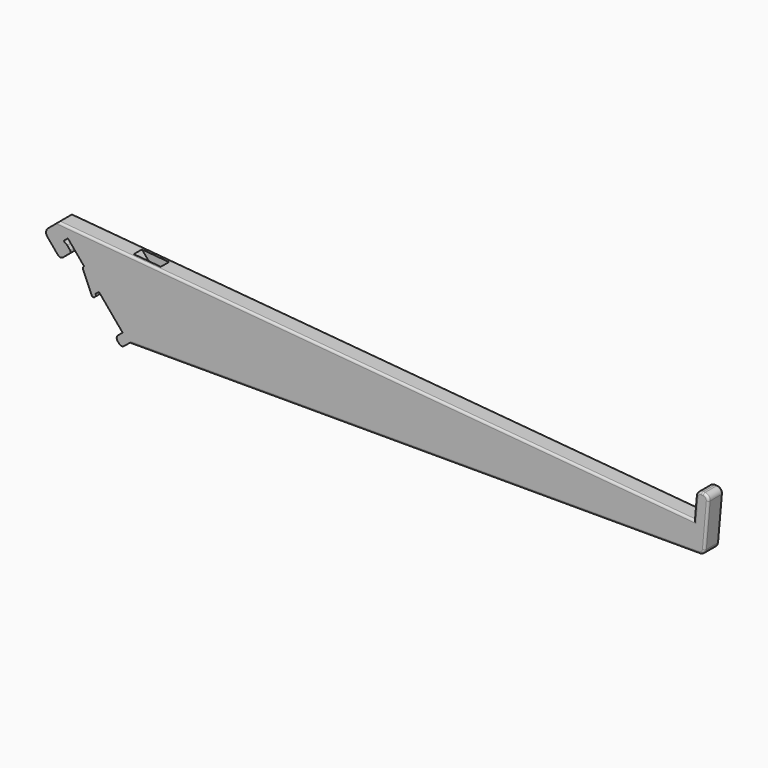
from build123d import *

# Parameters (mm, degrees)
F1_DEPTH = 12.7
F2_W     = 13.335
F2_H     = 7.112
F3_DEPTH = 93.472
F5_R     = 1.524


# Not quite as in the source:
# - two fillets or chamfers of one size are made in one step


with BuildPart() as f1:
    # F0 (on Front) → F1 (new body)
    with BuildSketch(Plane.XZ):
        with BuildLine():
            ThreePointArc((-46.0617865298, -15.3783926414), (-47.4082675367, -17.9649585898), (-46.5313950652, -20.7460427626))
            Line((-46.5313950652, -20.7460427626), (-39.1843326865, -29.5019307475))
            ThreePointArc((-39.1843326865, -29.5019307475), (-37.4599553875, -30.399584752), (-35.6058992724, -29.8150031044))
            Line((-35.6058992724, -29.8150031044), (-30.7415170586, -25.7333017829))
            ThreePointArc((-30.7415170586, -25.7333017829), (-30.2926900563, -24.8711131334), (-30.5849808801, -23.9440850758))
            Line((-30.5849808801, -23.9440850758), (-32.6258315409, -21.5118939689))
            Line((-32.6258315409, -21.5118939689), (-35.2214163384, -19.5451800716))
            Line((-35.2214163384, -19.5451800716), (-32.2344910947, -17.0388522013))
            Line((-32.2344910947, -17.0388522013), (-20.8873614209, -30.5618347556))
            Line((-20.8873614209, -30.5618347556), (-21.3737996423, -30.9700048878))
            ThreePointArc((-21.3737996423, -30.9700048878), (-21.7934146066, -31.6507945747), (-21.722945379, -32.4474032641))
            Line((-21.722945379, -32.4474032641), (-15.4658563045, -46.9017792559))
            ThreePointArc((-15.4658563045, -46.9017792559), (-14.603667655, -47.3506062582), (-13.6766395974, -47.0583154344))
            Line((-13.6766395974, -47.0583154344), (-12.2173249333, -45.8338050379))
            Line((-12.2173249333, -45.8338050379), (-13.0336651976, -44.8609285952))
            Line((-13.0336651976, -44.8609285952), (-10.6014740907, -42.8200779344))
            Line((-10.6014740907, -42.8200779344), (5.8885992482, -62.4721820782))
            Line((5.8885992482, -62.4721820782), (2.6781069871, -65.1661049504))
            ThreePointArc((2.6781069871, -65.1661049504), (1.7804529825, -66.8904822493), (2.3650346302, -68.7445383645))
            Line((2.3650346302, -68.7445383645), (3.4262769738, -70.0092777401))
            ThreePointArc((3.4262769738, -70.0092777401), (5.1506542727, -70.9069317447), (7.0047103879, -70.322350097))
            Line((7.0047103879, -70.322350097), (10.215202649, -67.6284272248))
            Line((10.215202649, -67.6284272248), (407.5256729651, -67.6284272248))
            ThreePointArc((407.5256729651, -67.6284272248), (410.0996716561, -66.6274538781), (411.3211747648, -64.1504906047))
            Line((411.3211747648, -64.1504906047), (413.9966944617, -33.5691605326))
            ThreePointArc((413.9966944617, -33.5691605326), (413.1198219902, -30.7880763598), (410.5332560418, -29.441595353))
            Line((410.5332560418, -29.441595353), (409.2680887752, -29.3309075597))
            ThreePointArc((409.2680887752, -29.3309075597), (406.4870046025, -30.2077800311), (405.1405235956, -32.7943459795))
            Line((405.1405235956, -32.7943459795), (403.8122700762, -47.9763531785))
            Line((403.8122700762, -47.9763531785), (-38.7652132091, -9.2558406592))
            Line((-38.7652132091, -9.2558406592), (-46.0617865298, -15.3783926414))
        make_face()
    extrude(amount=F1_DEPTH)

    # F2 (on face) → F3 (cut)
    with BuildSketch(Plane(origin=(-11.4592404683, 0, 13.6565909966), x_dir=(0.7660444431, 0, 0.6427876097), z_dir=(-0.6427876097, 0, 0.7660444431))):
        with Locations((6.6675, -6.35)):
            Rectangle(F2_W, F2_H)
    extrude(amount=-F3_DEPTH, mode=Mode.SUBTRACT)

    # F5
    f5_edges = [f1.edges().sort_by_distance(p)[0] for p in [
        (182.523528, 0, -28.616097),
        (404.476397, 0, -40.38535),
        (208.870438, 0, -67.628427),
        (409.900672, 0, -29.386251),
        (409.900672, -12.7, -29.386251),
        (413.119822, 0, -30.788076),
        (413.119822, -12.7, -30.788076),
        (406.487005, 0, -30.20778),
        (406.487005, -12.7, -30.20778),
        (410.099672, 0, -66.627454),
        (412.658935, 0, -48.859826),
        (404.476397, -12.7, -40.38535),
        (182.523528, -12.7, -28.616097),
        (208.870438, -12.7, -67.628427),
        (410.099672, -12.7, -66.627454),
        (412.658935, -12.7, -48.859826),
    ]]
    fillet(f5_edges, radius=F5_R)


solid = f1.part
